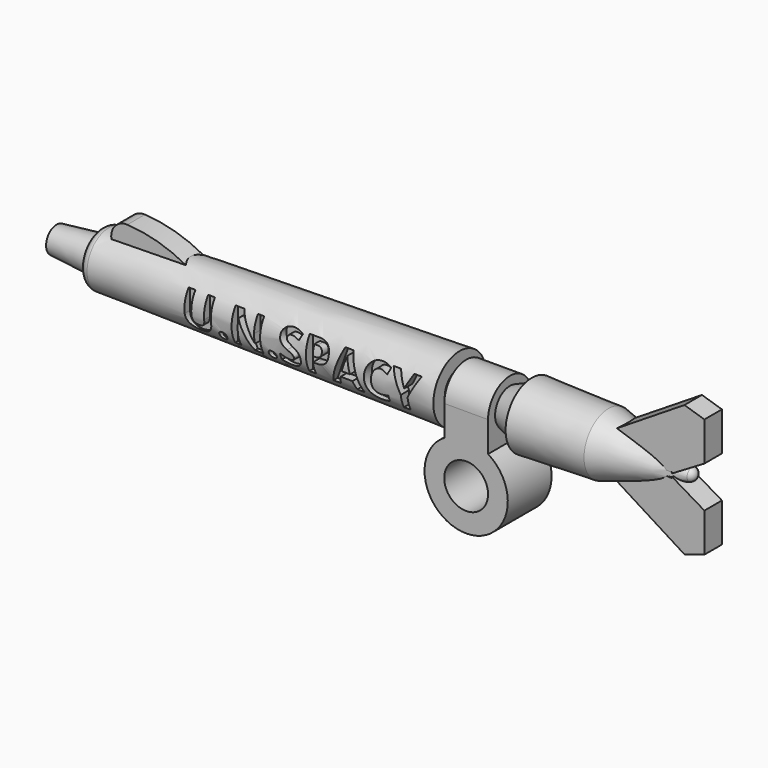
from build123d import *

# Parameters (mm, degrees)
F2_R         = 0.508
F4_DEPTH     = 0.635
F6_TEXT_SIZE = 2.6458333333
F7_DEPTH     = 25.4
F8_R         = 1.27
F9_DEPTH     = 1.5875


# Not quite as in the source:
# - Text() gives the source's letters only with a copy of the font that has no kerning and outlines rounded to 1/6400 em; it was checked with that copy


with BuildPart() as f1:
    # F0 (on Front) → F1 (revolve)
    with BuildSketch(Plane.XZ):
        with BuildLine():
            Line((-23.3655798899, 0.762), (-23.3655798899, 0))
            Line((-23.3655798899, 0), (13.7542079654, 0))
            ThreePointArc((13.7542079654, 0), (13.6779957721, 0.2286162569), (13.4798489476, 0.365771378))
            Line((13.4798489476, 0.365771378), (8.636, 1.778))
            Line((8.636, 1.778), (4.191, 1.905))
            Line((4.191, 1.905), (4.191, 1.5875))
            Line((4.191, 1.5875), (2.921, 1.0795))
            Line((2.921, 1.0795), (2.921, 1.5875))
            Line((2.921, 1.5875), (0.381, 1.5875))
            Line((0.381, 1.5875), (0.381, 1.0795))
            Line((0.381, 1.0795), (0, 1.0795))
            Line((0, 1.0795), (0, 1.905))
            Line((0, 1.905), (-20.8255798899, 1.5875))
            Line((-20.8255798899, 1.5875), (-20.8255798899, 1.016))
            Line((-20.8255798899, 1.016), (-23.3655798899, 0.762))
        make_face()
    revolve(axis=Axis((-4.8056859622, 0, 0), (-1, 0, 0)))

    # F2
    f2_edges = [f1.edges().sort_by_distance(p)[0] for p in [
        (-20.82558, 0, -1.5875),
    ]]
    fillet(f2_edges, radius=F2_R)

    # F3 (on Front) → F4 (join, symmetric)
    with BuildSketch(Plane.XZ):
        with BuildLine():
            ThreePointArc((-14.1660364199, 0.74081195), (-16.3190844683, 1.9929004313), (-18.7547452797, 2.5133789377))
            ThreePointArc((-18.7547452797, 2.5133789377), (-19.6878313093, 1.6921238484), (-18.887759355, 0.74081195))
            Line((-18.887759355, 0.74081195), (-14.1660364199, 0.74081195))
        make_face()
        Polygon((13.5427862406, 3.81), (8.9272540063, 0.9081602911), (12.4940136448, 0.0451405644), (12.4940136448, 0.1426670933), (12.8279812634, 0.1426670933), (12.8279812634, 0.0875470591), (14.7007163614, 1.199790803), (14.7007163614, 3.4506483935), align=None)
        Polygon((14.7007163614, -3.4506483935), (14.7007163614, -1.199790803), (12.8279812634, -0.0875470591), (12.8279812634, -0.1549278968), (12.4940136448, -0.1549278968), (12.4940136448, -0.0451405644), (8.9272540063, -0.9081602911), (13.5427862406, -3.81), align=None)
    extrude(amount=F4_DEPTH, both=True)

    # F6 (on offset) → F7 (cut)
    with BuildSketch(Plane.XZ.offset(1.27)):
        with Locations((-14.8337301381, -0.9210634108)):
            Text('U.N.SPACY', F6_TEXT_SIZE, font='Open Sans', font_style=FontStyle.BOLD, text_align=(TextAlign.LEFT, TextAlign.BOTTOM))
    extrude(amount=F7_DEPTH, mode=Mode.SUBTRACT)

    # F8 (on Front) → F9 (join, symmetric)
    with BuildSketch(Plane.XZ):
        with BuildLine():
            Line((2.921, 0), (0.381, 0))
            Line((0.381, 0), (0.381, -1.7582522085))
            ThreePointArc((0.381, -1.7582522085), (1.651, -6.223), (2.921, -1.7582522085))
            Line((2.921, -1.7582522085), (2.921, 0))
        make_face()
        with Locations((1.651, -3.81)):
            Circle(F8_R, mode=Mode.SUBTRACT)
    extrude(amount=F9_DEPTH, both=True)


solid = f1.part
